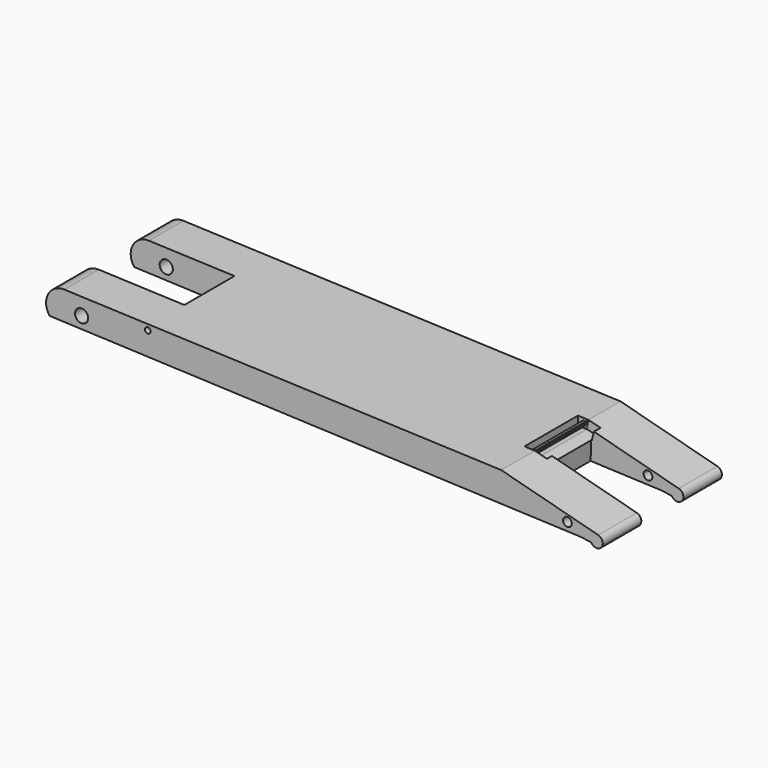
from build123d import *

# Parameters (mm, degrees)
F1_DEPTH      = 85
F2_W          = 140.1526774555
F2_H          = 71.5
F2_W_2        = 166.0307588987
F2_H_2        = 60
F3_DEPTH      = 60
F4_R          = 5
F5_DEPTH      = 115.001
F5_DEPTH_BACK = 55.001
F6_R          = 7.5
F7_DEPTH      = 120.751
F7_DEPTH_BACK = 49.251
F8_W          = 2.8015428152
F8_H          = 60
F9_DEPTH      = 10
F11_W         = 11.8633863517
F11_H         = 76.3498097658
F12_DEPTH     = 10
F13_R         = 2.5
F14_DEPTH     = 76.3498097658
F15_R         = 3.25
F16_DEPTH     = 20


# Not quite as in the source:
# - a feature of the source that left no trace in its solid (it failed there, or was rolled back) is left out
# - a feature names something its author has since deleted; it is built from what else it names


with BuildPart() as f1:
    # F0 (on Front) → F1 (new body, symmetric)
    with BuildSketch(Plane.XZ):
        with BuildLine():
            Line((279.3908679786, 0.7735525745), (-219.4691173488, 19.9851854498))
            ThreePointArc((-219.4691173488, 19.9851854498), (-237.9331597041, 9.3224734741), (-236.2868942017, -11.9355625752))
            Line((-236.2868942017, -11.9355625752), (370.8640205953, -36.8868572182))
            Line((370.8640205953, -36.8868572182), (382.0565363882, -38.6184028055))
            ThreePointArc((382.0565363882, -38.6184028055), (393.7122397041, -39.6064498563), (390.0009393692, -28.5133030266))
            Line((390.0009393692, -28.5133030266), (279.3908679786, 0.7735525745))
        make_face()
    extrude(amount=F1_DEPTH, both=True)

    # F2 (on face) → F3 (cut)
    with BuildSketch(Plane(origin=(0.44349793, 0, 11.5161148616), x_dir=(0.9992592725, 0, -0.0384825459), z_dir=(0.0384825459, 0, 0.9992592725))):
        with Locations((-192.4187466502, 0)):
            Rectangle(F2_W, F2_H)
        with Locations((373.3601896558, 0)):
            Rectangle(F2_W_2, F2_H_2)
    extrude(amount=-F3_DEPTH, mode=Mode.SUBTRACT)

    # F4 (on face) → F5 (cut, two sides)
    with BuildSketch(Plane(origin=(0, -30, 0), x_dir=(-1, 0, 0), z_dir=(0, 1, 0))) as f5_sk:
        with Locations((-354.8175990582, -26.7948582768)):
            Circle(F4_R)
    extrude(amount=F5_DEPTH, mode=Mode.SUBTRACT)
    extrude(f5_sk.sketch, amount=-F5_DEPTH_BACK, mode=Mode.SUBTRACT)

    # F6 (on face) → F7 (cut, two sides)
    with BuildSketch(Plane.XZ.offset(-35.75)) as f7_sk:
        with Locations((-199.6834129095, 0)):
            Circle(F6_R)
    extrude(amount=F7_DEPTH, mode=Mode.SUBTRACT)
    extrude(f7_sk.sketch, amount=-F7_DEPTH_BACK, mode=Mode.SUBTRACT)

    # F8 (on face) → F9 (cut)
    with BuildSketch(Plane(origin=(18.495209297, 0, 69.8523750243), x_dir=(0.9666885377, 0, -0.2559556038), z_dir=(0.2559556038, 0, 0.9666885377))):
        Polygon((270.5007791519, -37.1644198895), (284.1554284096, -37.1644198895), (284.1554284096, -30), (281.3538855944, -30), (281.3538855944, 30), (284.1554284096, 30), (284.1554284096, 39.305575192), (270.5007791519, 39.305575192), align=None)
        with Locations((282.754657002, 0)):
            Rectangle(F8_W, F8_H)
    extrude(amount=-F9_DEPTH, mode=Mode.SUBTRACT)

    # F11 (on face) → F12 (cut)
    with BuildSketch(Plane(origin=(0.44349793, 0, 11.5161148616), x_dir=(0.9992592725, 0, -0.0384825459), z_dir=(0.0384825459, 0, 0.9992592725))):
        with Locations((273.2224540287, 1.0649263859)):
            Rectangle(F11_W, F11_H)
    extrude(amount=-F12_DEPTH, mode=Mode.SUBTRACT)

    # F13 (on face) → F14 (join, through all)
    with BuildSketch(Plane.XZ.offset(-39.2398312688)):
        with Locations((274.223446846, -4.3092062697)):
            Circle(F13_R)
    extrude(amount=F14_DEPTH)

    # F15 (on face) → F16 (cut)
    with BuildSketch(Plane.XZ.offset(85)):
        with Locations((-124.1565719247, 9.9523849785)):
            Circle(F15_R)
    extrude(amount=-F16_DEPTH, mode=Mode.SUBTRACT)


solid = f1.part
